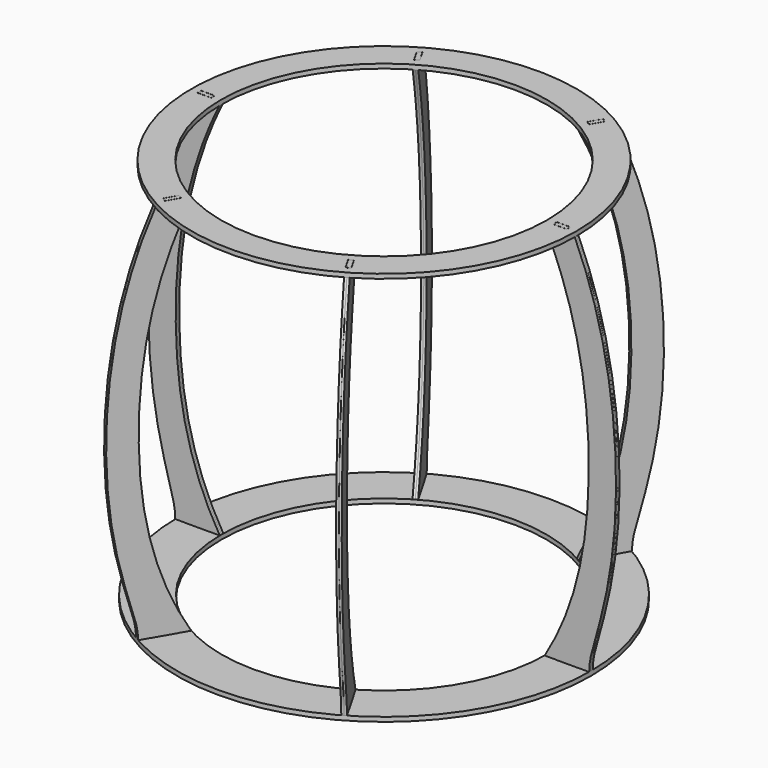
from build123d import *

# Parameters (mm, degrees)
F0_W     = 76.2
F0_H     = 25.4
F0_W_2   = 127
F1_DEPTH = 12.7
F2_COUNT = 6
F4_R     = 1181.8412542343
F4_W     = 128.27
F4_H     = 26.67
F4_R_2   = 927.8412542343
F5_DEPTH = 25.4
F7_R     = 1099.6887199782
F7_W     = 77.47
F7_H     = 26.67
F7_R_2   = 930.9359849962
F8_DEPTH = 25.4


with BuildPart() as f1:
    # F0 (on Front) → F1 (new body, symmetric)
    with BuildSketch(Plane.XZ):
        with BuildLine():
            add(Edge.make_bspline(
                [(-1099.6887199782, 1008.0922653193), (-1100.0337344398, 1007.3338657486), (-1329.3225968452, 502.576775956), (-1377.2601767834, -395.2960237062), (-1222.9775693795, -953.8734029081), (-1181.8412542343, -1091.579079628), (-1181.8412542343, -1150.9077346807)],
                knots=[0.3364637021, 0.3364637021, 0.3364637021, 0.3364637021, 0.3369736623, 0.675814076, 0.8805104312, 1, 1, 1, 1], degree=3))
            Line((-1181.8412542343, -1150.9077346807), (-1118.3412542343, -1150.9077346807))
            Line((-1118.3412542343, -1150.9077346807), (-1118.3412542343, -1125.5077346807))
            Line((-1118.3412542343, -1125.5077346807), (-991.3412542343, -1125.5077346807))
            Line((-991.3412542343, -1125.5077346807), (-991.3412542343, -1150.9077346807))
            Line((-991.3412542343, -1150.9077346807), (-927.8412542343, -1150.9077346807))
            add(Edge.make_bspline(
                [(-927.8412542343, -1150.9077346807), (-1116.0754534599, -839.7431185847), (-1243.5716770375, -126.3422574808), (-1114.0437083882, 637.5344643087), (-930.9359849962, 1008.0922653193)],
                knots=[0.2469302761, 0.2469302761, 0.2469302761, 0.2469302761, 0.4876340437, 0.7376984774, 0.7376984774, 0.7376984774, 0.7376984774], degree=3))
            Line((-930.9359849962, 1008.0922653193), (-977.2123524872, 1008.0922653193))
            Line((-977.2123524872, 1008.0922653193), (-977.2123524872, 982.6922653193))
            Line((-977.2123524872, 982.6922653193), (-1053.4123524872, 982.6922653193))
            Line((-1053.4123524872, 982.6922653193), (-1053.4123524872, 1008.0922653193))
            Line((-1053.4123524872, 1008.0922653193), (-1099.6887199782, 1008.0922653193))
        make_face()
        with Locations((-1015.3123524872, 995.3922653193)):
            Rectangle(F0_W, F0_H)
        with Locations((-1015.3123524872, 1020.7922653193)):
            Rectangle(F0_W, F0_H)
        with Locations((-1054.8412542343, -1138.2077346807)):
            Rectangle(F0_W_2, F0_H)
        with Locations((-1054.8412542343, -1163.6077346807)):
            Rectangle(F0_W_2, F0_H)
    extrude(amount=F1_DEPTH, both=True)


with BuildPart() as f2_1:
    # F2: instance of F1
    add(f1.part.rotate(Axis((0, 0, 1876.9995654606), (0, 0, -1)), 1 * 360 / F2_COUNT))


with BuildPart() as f2_2:
    # F2: instance of F1
    add(f1.part.rotate(Axis((0, 0, 1876.9995654606), (0, 0, -1)), 2 * 360 / F2_COUNT))


with BuildPart() as f2_3:
    # F2: instance of F1
    add(f1.part.rotate(Axis((0, 0, 1876.9995654606), (0, 0, -1)), 3 * 360 / F2_COUNT))


with BuildPart() as f2_4:
    # F2: instance of F1
    add(f1.part.rotate(Axis((0, 0, 1876.9995654606), (0, 0, -1)), 4 * 360 / F2_COUNT))


with BuildPart() as f2_5:
    # F2: instance of F1
    add(f1.part.rotate(Axis((0, 0, 1876.9995654606), (0, 0, -1)), 5 * 360 / F2_COUNT))


with BuildPart() as f5:
    # F4 (on face) → F5 (new body)
    with BuildSketch(Plane.XY.offset(-1150.9077346807)):
        Circle(F4_R)
        Polygon((-547.9396783577, -975.7293623985), (-571.0365758766, -962.3943623985), (-506.9015758766, -851.309283855), (-483.8046783577, -864.644283855), align=None, mode=Mode.SUBTRACT)
        Polygon((571.0365758766, -962.3943623985), (547.9396783577, -975.7293623985), (483.8046783577, -864.644283855), (506.9015758766, -851.309283855), align=None, mode=Mode.SUBTRACT)
        with Locations((-1054.8412542343, 0)):
            Rectangle(F4_W, F4_H, mode=Mode.SUBTRACT)
        Polygon((-571.0365758766, 962.3943623985), (-547.9396783577, 975.7293623985), (-483.8046783577, 864.644283855), (-506.9015758766, 851.309283855), align=None, mode=Mode.SUBTRACT)
        Circle(F4_R_2, mode=Mode.SUBTRACT)
        with Locations((1054.8412542343, 0)):
            Rectangle(F4_W, F4_H, mode=Mode.SUBTRACT)
        Polygon((547.9396783577, 975.7293623985), (571.0365758766, 962.3943623985), (506.9015758766, 851.309283855), (483.8046783577, 864.644283855), align=None, mode=Mode.SUBTRACT)
    extrude(amount=-F5_DEPTH)


with BuildPart() as f8:
    # F7 (on plane+point) → F8 (new body)
    with BuildSketch(Plane.XY.offset(1008.0922653193)):
        Circle(F7_R)
        Polygon((-515.4752274841, -919.4992840457), (-538.5721250031, -906.1642840457), (-499.8371250031, -839.0732960145), (-476.7402274841, -852.4082960145), align=None, mode=Mode.SUBTRACT)
        Polygon((538.5721250031, -906.1642840457), (515.4752274841, -919.4992840457), (476.7402274841, -852.4082960145), (499.8371250031, -839.0732960145), align=None, mode=Mode.SUBTRACT)
        with Locations((-1015.3123524872, 0)):
            Rectangle(F7_W, F7_H, mode=Mode.SUBTRACT)
        Polygon((-538.5721250031, 906.1642840457), (-515.4752274841, 919.4992840457), (-476.7402274841, 852.4082960145), (-499.8371250031, 839.0732960145), align=None, mode=Mode.SUBTRACT)
        Circle(F7_R_2, mode=Mode.SUBTRACT)
        with Locations((1015.3123524872, 0)):
            Rectangle(F7_W, F7_H, mode=Mode.SUBTRACT)
        Polygon((515.4752274841, 919.4992840457), (538.5721250031, 906.1642840457), (499.8371250031, 839.0732960145), (476.7402274841, 852.4082960145), align=None, mode=Mode.SUBTRACT)
    extrude(amount=F8_DEPTH)


solid = Compound([f1.part, f2_1.part, f2_2.part, f2_3.part, f2_4.part, f2_5.part, f5.part, f8.part])
